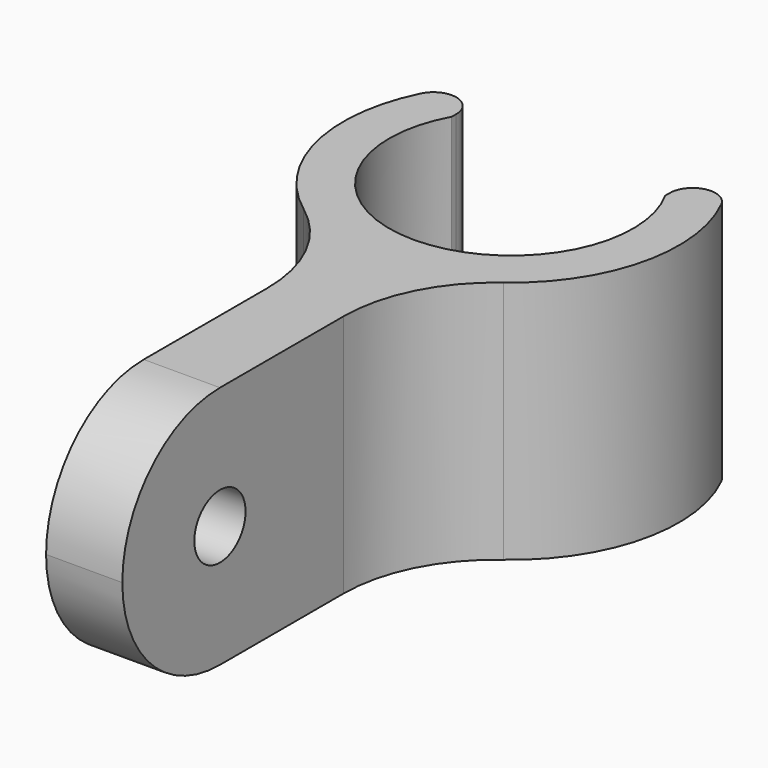
from build123d import *

# Parameters (mm, degrees)
F0_R     = 8
F1_DEPTH = 16
F3_DEPTH = 25
F4_R     = 1.5
F5_R     = 7.99999
F6_R     = 10
F7_R     = 2.1
F8_DEPTH = 25


# Not quite as in the source:
# - a fillet or chamfer is up to 0.001 mm smaller than in the source, because OpenCascade refuses the exact size


with BuildPart() as f1:
    # F0 (on Top) → F1 (new body)
    with BuildSketch(Plane.XY):
        with BuildLine():
            Line((2.5, -35), (2.5, -10.7121426428))
            ThreePointArc((2.5, -10.7121426428), (0, 11), (-2.5, -10.7121426428))
            Line((-2.5, -10.7121426428), (-2.5, -35))
            Line((-2.5, -35), (2.5, -35))
        make_face()
        Circle(F0_R, mode=Mode.SUBTRACT)
    extrude(amount=F1_DEPTH)

    # F2 (on face) → F3 (cut)
    with BuildSketch(Plane.XY.offset(16)):
        with BuildLine():
            ThreePointArc((-7, 3.8729833462), (0, 8), (7, 3.8729833462))
            Line((7, 3.8729833462), (7, 8.4852813742))
            ThreePointArc((7, 8.4852813742), (0, 11), (-7, 8.4852813742))
            Line((-7, 8.4852813742), (-7, 3.8729833462))
        make_face()
    extrude(amount=-F3_DEPTH, mode=Mode.SUBTRACT)

    # F4
    f4_edges = [f1.edges().sort_by_distance(p)[0] for p in [
        (-7, 8.485281, 8),
        (7, 8.485281, 8),
    ]]
    fillet(f4_edges, radius=F4_R)

    # F5 (radius 8 in the source; OpenCascade refuses exactly that, so slightly less here)
    f5_edges = [f1.edges().sort_by_distance(p)[0] for p in [
        (0, -35, 16),
        (0, -35, 0),
    ]]
    fillet(f5_edges, radius=F5_R)

    # F6
    f6_edges = [f1.edges().sort_by_distance(p)[0] for p in [
        (-2.5, -10.712143, 8),
        (2.5, -10.712143, 8),
    ]]
    fillet(f6_edges, radius=F6_R)

    # F7 (on face) → F8 (cut)
    with BuildSketch(Plane(origin=(-2.5, 0, 0), x_dir=(0, -1, 0), z_dir=(-1, 0, 0))):
        with Locations((27, 8)):
            Circle(F7_R)
    extrude(amount=-F8_DEPTH, mode=Mode.SUBTRACT)


solid = f1.part
